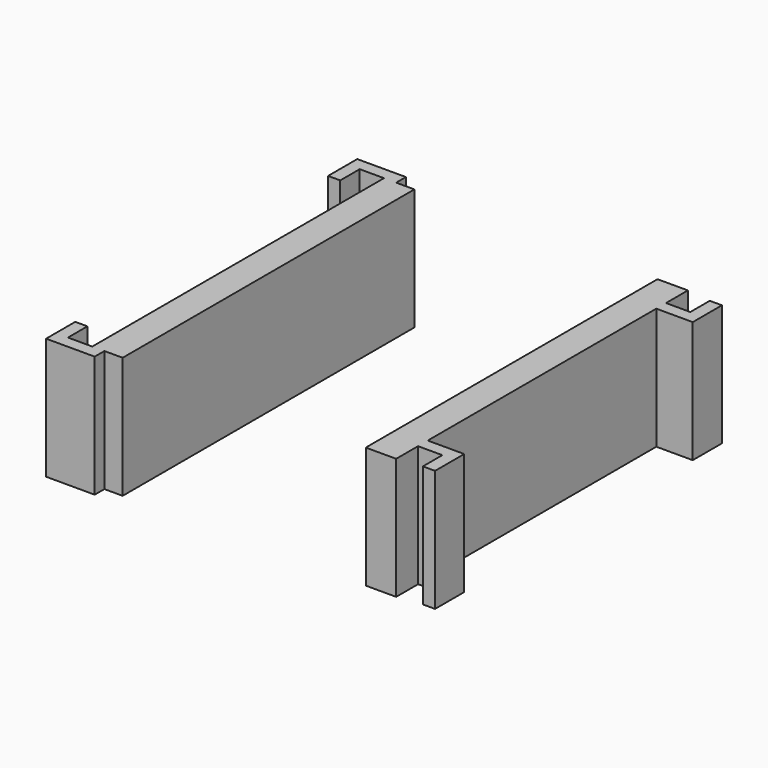
from build123d import *

# Parameters (mm, degrees)
F0_W     = 5
F0_H     = 47
F0_W_2   = 2
F0_H_2   = 4
F0_H_3   = 2
F1_DEPTH = 20
F0_W_3   = 4


with BuildPart() as f1:
    # F0 (on Top) → F1 (new body)
    with BuildSketch(Plane.XY):
        Polygon((-29, 30), (-25, 30), (-23, 30), (-23, 32), (-29, 32), align=None)
        Polygon((-23, 30), (-25, 30), (-25, 23.5), (-20, 23.5), (-20, 30), align=None)
        with Locations((-22.5, 0)):
            Rectangle(F0_W, F0_H)
        with Locations((-30, 28)):
            Rectangle(F0_W_2, F0_H_2)
        with Locations((-30, 31)):
            Rectangle(F0_W_2, F0_H_3)
        Polygon((-20, -23.5), (-25, -23.5), (-25, -30), (-23, -30), (-20, -30), align=None)
        Polygon((-23, -30), (-25, -30), (-29, -30), (-29, -32), (-23, -32), align=None)
        with Locations((-30, -31)):
            Rectangle(F0_W_2, F0_H_3)
        with Locations((-30, -28)):
            Rectangle(F0_W_2, F0_H_2)
    extrude(amount=F1_DEPTH)


with BuildPart() as f1b:
    # F0 (on Top) → F1, piece 2 (new body)
    with BuildSketch(Plane.XY):
        Polygon((25, 30), (20, 30), (20, 23.5), (25, 23.5), (25, 25.5), align=None)
        with Locations((22.5, 0)):
            Rectangle(F0_W, F0_H)
        Polygon((25, -23.5), (20, -23.5), (20, -30), (25, -30), (25, -25.5), align=None)
        with Locations((27, 24.5)):
            Rectangle(F0_W_3, F0_H_3)
        with Locations((27, -24.5)):
            Rectangle(F0_W_3, F0_H_3)
        Polygon((29, 25.5), (29, 23.5), (31, 23.5), (31, 29.5), (29, 29.5), align=None)
        Polygon((31, -23.5), (29, -23.5), (29, -25.5), (29, -29.5), (31, -29.5), align=None)
    extrude(amount=F1_DEPTH)


solid = Compound([f1.part, f1b.part])
